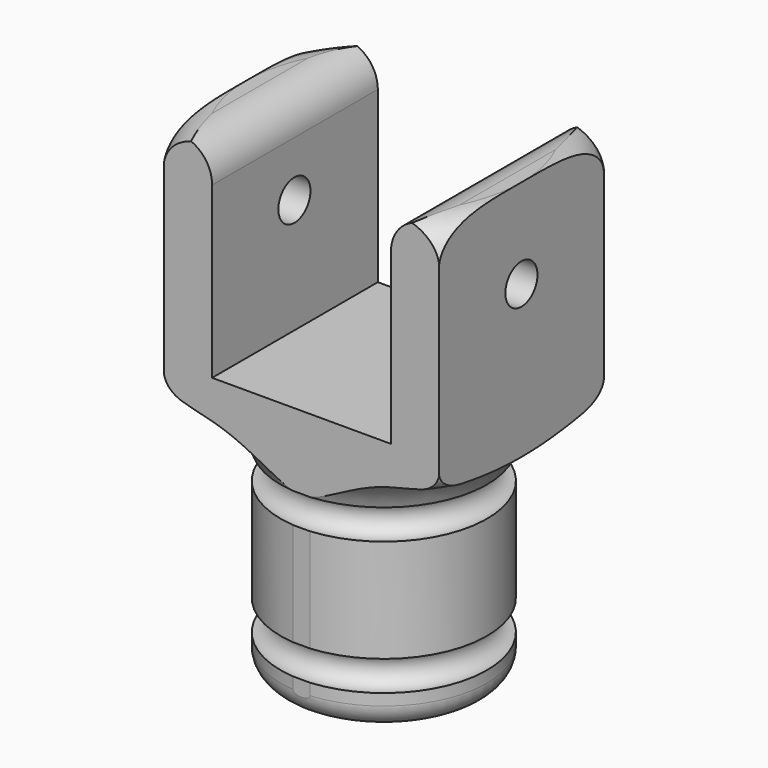
from build123d import *

# Parameters (mm, degrees)
F2_W         = 15.6
F2_H         = 18
F3_DEPTH     = 20
F4_R         = 1.75
F5_DEPTH     = 25
F6_R         = 2
F8_T4_ANGLE  = 85.6888117938
F8_T10_ANGLE = 85.6888117938
F9_R         = 3
F10_W        = 18.064645119
F10_H        = 45.2089011669
F11_DEPTH    = 12


# Not quite as in the source:
# - a fillet or chamfer that OpenCascade refuses, or shapes differently, is made with other operations: its cross-section is extruded or revolved along the edge and cut away or added


with BuildPart() as f1:
    # F0 (on Front) → F1 (revolve)
    with BuildSketch(Plane.XZ):
        with BuildLine():
            Line((0, 20), (-15, 20))
            Line((-15, 20), (-15, 0))
            Line((-15, 0), (-9, -2.1838214056))
            Line((-9, -2.1838214056), (-9, -4.1838214056))
            ThreePointArc((-9, -4.1838214056), (-7.5, -5.4972139593), (-9, -6.8106065129))
            Line((-9, -6.8106065129), (-9, -15.8106065129))
            ThreePointArc((-9, -15.8106065129), (-7.5, -17.1239990666), (-9, -18.4373916202))
            Line((-9, -18.4373916202), (-9, -21.4373916202))
            Line((-9, -21.4373916202), (-1, -21.4373916202))
            Line((-1, -21.4373916202), (-1, -20.3507256404))
            Line((-1, -20.3507256404), (-5.5, -18.6372557045))
            Line((-5.5, -18.6372557045), (-5.5, -2.1838214056))
            Line((-5.5, -2.1838214056), (0, 0))
            Line((0, 0), (0, 20))
        make_face()
    revolve(axis=Axis((0, 0, 10), (0, 0, 1)))

    # F2 (on Front) → F3 (cut, symmetric)
    with BuildSketch(Plane.XZ):
        with Locations((0, 11.1958423193)):
            Rectangle(F2_W, F2_H)
    extrude(amount=F3_DEPTH, both=True, mode=Mode.SUBTRACT)

    # F4 (on face) → F5 (cut, symmetric)
    with BuildSketch(Plane(origin=(7.8, 0, 0), x_dir=(0, -1, 0), z_dir=(-1, 0, 0))):
        with Locations((0, 12.1958423193)):
            Circle(F4_R)
    extrude(amount=F5_DEPTH, both=True, mode=Mode.SUBTRACT)

    # F6
    f6_edges = [f1.edges().sort_by_distance(p)[0] for p in [
        (9, 0, -21.437392),
        (15, 0, 0),
    ]]
    fillet(f6_edges, radius=F6_R)

    # F7: fillet of radius 5 on 1 edges, made by hand

    # F7_s1 → F7_t2 (revolve)
    with BuildSketch(Plane.XZ):
        with BuildLine():
            ThreePointArc((-9, -4.1838214056), (-10.1604252956, -2.2874600731), (-12.0282444437, -1.081630566))
            Line((-12.0282444437, -1.081630566), (-11.9940424293, -0.9876613039))
            Line((-11.9940424293, -0.9876613039), (-8.9657979857, -2.0898521435))
            Line((-8.9657979857, -2.0898521435), (-8.9, -2.1838214056))
            ThreePointArc((-8.9, -2.1838214056), (-8.9, -3.1838214056), (-8.9052330968, -4.1518959603))
            Line((-8.9052330968, -4.1518959603), (-9, -4.1838214056))
        make_face()
    revolve(axis=Axis((0, 0, -2.1838214056), (0, 0, 1)))

    # F8: fillet of radius 1 on 2 edges, made by hand


with BuildPart() as f8_tool2:
    # F8_s3 → F8_t4 (revolve)
    with BuildSketch(Plane(origin=(0, 0, 0), x_dir=(0, 0, 1), z_dir=(-0.7332030574, -0.6800097621, 0))):
        with BuildLine():
            ThreePointArc((0.9912700225, 14.9576852568), (1.8264879025, 14.7549047682), (2.1958423193, 13.9788337995))
            Line((2.1958423193, 13.9788337995), (2.2958423193, 13.9788337995))
            Line((2.2958423193, 13.9788337995), (2.2958423193, 15))
            Line((2.2958423193, 15), (2.1958423193, 15.1))
            ThreePointArc((2.1958423193, 15.1), (1.4004150764, 15.0999823888), (0.9708127928, 15.0555704025))
            Line((0.9708127928, 15.0555704025), (0.9912700225, 14.9576852568))
        make_face()
    revolve(axis=Axis((0, 0, 2.1958423193), (0, 0, -1)), revolution_arc=F8_T4_ANGLE)

    split(bisect_by=Plane.YZ.offset(-7.8), keep=Keep.TOP)

    split(bisect_by=Plane.YZ.offset(7.8), keep=Keep.BOTTOM)


with BuildPart() as f1_1:
    add(f1.part)

    # F8_t1: cut F8_tool2
    add(f8_tool2.part, mode=Mode.SUBTRACT)


with BuildPart() as f8_tool8:
    # F8_s9 → F8_t10 (revolve)
    with BuildSketch(Plane(origin=(0, 0, 0), x_dir=(0, 0, 1), z_dir=(0.7332030574, 0.6800097621, 0))):
        with BuildLine():
            ThreePointArc((0.9912700225, 14.9576852568), (1.8264879025, 14.7549047682), (2.1958423193, 13.9788337995))
            Line((2.1958423193, 13.9788337995), (2.2958423193, 13.9788337995))
            Line((2.2958423193, 13.9788337995), (2.2958423193, 15))
            Line((2.2958423193, 15), (2.1958423193, 15.1))
            ThreePointArc((2.1958423193, 15.1), (1.4004150764, 15.0999823888), (0.9708127928, 15.0555704025))
            Line((0.9708127928, 15.0555704025), (0.9912700225, 14.9576852568))
        make_face()
    revolve(axis=Axis((0, 0, 2.1958423193), (0, 0, -1)), revolution_arc=F8_T10_ANGLE)

    split(bisect_by=Plane.YZ.offset(-7.8), keep=Keep.TOP)

    split(bisect_by=Plane.YZ.offset(7.8), keep=Keep.BOTTOM)


with BuildPart() as f1_2:
    add(f1_1.part)

    # F8_t7: cut F8_tool8
    add(f8_tool8.part, mode=Mode.SUBTRACT)

    # F9
    f9_edges = [f1_2.edges().sort_by_distance(p)[0] for p in [
        (-7.8, 0, 20),
        (-15, 0, 20),
        (7.8, 0, 20),
        (15, 0, 20),
    ]]
    fillet(f9_edges, radius=F9_R)

    # F10 (on Right) → F11 (intersect, symmetric)
    with BuildSketch(Plane.YZ):
        with Locations((0.0636042096, 0.2437252551)):
            Rectangle(F10_W, F10_H)
    extrude(amount=F11_DEPTH, both=True, mode=Mode.INTERSECT)


solid = f1_2.part
